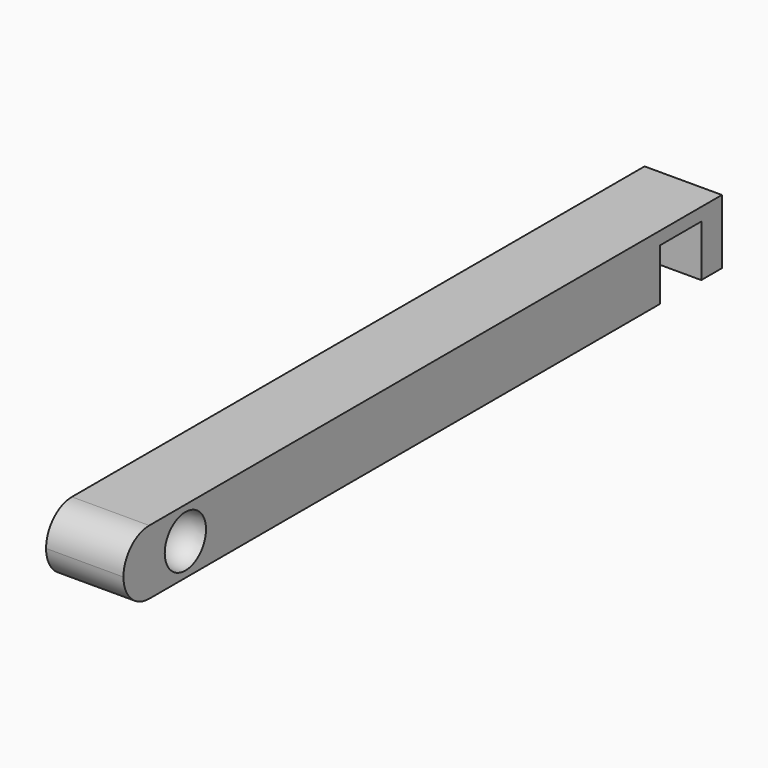
from build123d import *

# Parameters (mm, degrees)
F0_W     = 3
F0_H     = 29
F1_DEPTH = 2.5
F6_R     = 1.24999
F7_W     = 3
F7_H     = 2
F8_DEPTH = 2


# Not quite as in the source:
# - a fillet or chamfer is up to 0.001 mm smaller than in the source, because OpenCascade refuses the exact size


with BuildPart() as f1:
    # F0 (on Top) → F1 (new body)
    with BuildSketch(Plane.XY):
        with Locations((-28.6103483079, 8.1154592335)):
            Rectangle(F0_W, F0_H)
    extrude(amount=F1_DEPTH)

    # F2 (on face) → F3 (revolve, cut)
    with BuildSketch(Plane.YZ.offset(-27.1103483079)):
        with BuildLine():
            Line((-3.3845407665, 0.25), (-3.3845407665, 2.25))
            ThreePointArc((-3.3845407665, 2.25), (-4.3845407665, 1.25), (-3.3845407665, 0.25))
        make_face()
    revolve(axis=Axis((-27.1103483079, -3.3845407665, 1.25), (0, 0, -1)), mode=Mode.SUBTRACT)

    # F4 (on face) → F5 (revolve, cut)
    with BuildSketch(Plane(origin=(-30.1103483079, 0, 0), x_dir=(0, -1, 0), z_dir=(-1, 0, 0))):
        with BuildLine():
            Line((2.3845407665, 1.25), (4.3845407665, 1.25))
            ThreePointArc((4.3845407665, 1.25), (3.3845407665, 2.25), (2.3845407665, 1.25))
        make_face()
    revolve(axis=Axis((-30.1103483079, -3.3845407665, 1.25), (0, -1, 0)), mode=Mode.SUBTRACT)

    # F6 (radius 1.25 in the source; OpenCascade refuses exactly that, so slightly less here)
    f6_edges = [f1.edges().sort_by_distance(p)[0] for p in [
        (-28.610348, -6.384541, 2.5),
        (-28.610348, -6.384541, 0),
    ]]
    fillet(f6_edges, radius=F6_R)

    # F7 (on face) → F8 (cut)
    with BuildSketch(Plane(origin=(0, 0, 0), x_dir=(1, 0, 0), z_dir=(0, 0, -1))):
        with Locations((-28.6103483079, -20.6154592335)):
            Rectangle(F7_W, F7_H)
    extrude(amount=-F8_DEPTH, mode=Mode.SUBTRACT)


solid = f1.part
